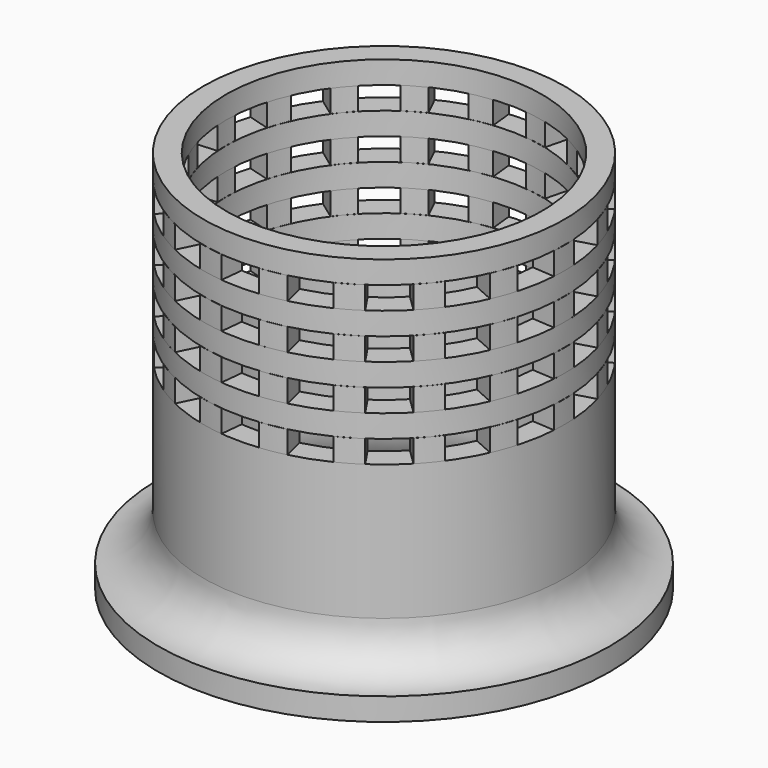
from build123d import *

# Parameters (mm, degrees)
F0_W          = 5
F0_H          = 30
F0_H_2        = 5
F2_ANGLE_BACK = 4
F2_ANGLE      = 8
F3_COUNT      = 18


# Not quite as in the source:
# - a feature names something its author has since deleted; it is built from what else it names


with BuildPart() as f1:
    # F0 (on Front) → F1 (revolve)
    with BuildSketch(Plane.XZ):
        with Locations((-37.5, 15)):
            Rectangle(F0_W, F0_H)
        with BuildLine():
            Line((-35, 0), (-40, 0))
            ThreePointArc((-40, 0), (-42.9289321881, -7.0710678119), (-50, -10))
            Line((-50, -10), (-50, -15))
            ThreePointArc((-50, -15), (-39.3933982822, -10.6066017178), (-35, 0))
        make_face()
    revolve(axis=Axis((0, 0, 67.5), (0, 0, -1)))


with BuildPart() as f1b:
    # F0 (on Front) → F1, piece 2 (revolve)
    with BuildSketch(Plane.XZ):
        with Locations((-37.5, 37.5)):
            Rectangle(F0_W, F0_H_2)
    revolve(axis=Axis((0, 0, 67.5), (0, 0, -1)))


with BuildPart() as f1c:
    # F0 (on Front) → F1, piece 3 (revolve)
    with BuildSketch(Plane.XZ):
        with Locations((-37.5, 47.5)):
            Rectangle(F0_W, F0_H_2)
    revolve(axis=Axis((0, 0, 67.5), (0, 0, -1)))


with BuildPart() as f1d:
    # F0 (on Front) → F1, piece 4 (revolve)
    with BuildSketch(Plane.XZ):
        with Locations((-37.5, 57.5)):
            Rectangle(F0_W, F0_H_2)
    revolve(axis=Axis((0, 0, 67.5), (0, 0, -1)))


with BuildPart() as f1e:
    # F0 (on Front) → F1, piece 5 (revolve)
    with BuildSketch(Plane.XZ):
        with Locations((-37.5, 67.5)):
            Rectangle(F0_W, F0_H_2)
    revolve(axis=Axis((0, 0, 67.5), (0, 0, -1)))


with BuildPart() as f2:
    # F0 (on Front) → F2 (revolve)
    with BuildSketch(Plane.XZ, mode=Mode.PRIVATE) as f2_sk:
        with Locations((-37.5, 42.5)):
            Rectangle(F0_W, F0_H_2)
    revolve(f2_sk.sketch.rotate(Axis((0, 0, 67.5), (0, 0, -1)), -F2_ANGLE_BACK), axis=Axis((0, 0, 67.5), (0, 0, -1)), revolution_arc=F2_ANGLE)


with BuildPart() as f2b:
    # F0 (on Front) → F2, piece 2 (revolve)
    with BuildSketch(Plane.XZ, mode=Mode.PRIVATE) as f2_sk:
        with Locations((-37.5, 52.5)):
            Rectangle(F0_W, F0_H_2)
    revolve(f2_sk.sketch.rotate(Axis((0, 0, 67.5), (0, 0, -1)), -F2_ANGLE_BACK), axis=Axis((0, 0, 67.5), (0, 0, -1)), revolution_arc=F2_ANGLE)


with BuildPart() as f2c:
    # F0 (on Front) → F2, piece 3 (revolve)
    with BuildSketch(Plane.XZ, mode=Mode.PRIVATE) as f2_sk:
        with Locations((-37.5, 62.5)):
            Rectangle(F0_W, F0_H_2)
    revolve(f2_sk.sketch.rotate(Axis((0, 0, 67.5), (0, 0, -1)), -F2_ANGLE_BACK), axis=Axis((0, 0, 67.5), (0, 0, -1)), revolution_arc=F2_ANGLE)


with BuildPart() as f2d:
    # F0 (on Front) → F2, piece 4 (revolve)
    with BuildSketch(Plane.XZ, mode=Mode.PRIVATE) as f2_sk:
        with Locations((-37.5, 32.5)):
            Rectangle(F0_W, F0_H_2)
    revolve(f2_sk.sketch.rotate(Axis((0, 0, 67.5), (0, 0, -1)), -F2_ANGLE_BACK), axis=Axis((0, 0, 67.5), (0, 0, -1)), revolution_arc=F2_ANGLE)


with BuildPart() as f3_1:
    # F3: instance of F2c
    add(f2c.part.rotate(Axis((0, 0, 67.5), (0, 0, -1)), 1 * 360 / F3_COUNT))


with BuildPart() as f3_2:
    # F3: instance of F2c
    add(f2c.part.rotate(Axis((0, 0, 67.5), (0, 0, -1)), 2 * 360 / F3_COUNT))


with BuildPart() as f3_3:
    # F3: instance of F2c
    add(f2c.part.rotate(Axis((0, 0, 67.5), (0, 0, -1)), 3 * 360 / F3_COUNT))


with BuildPart() as f3_4:
    # F3: instance of F2c
    add(f2c.part.rotate(Axis((0, 0, 67.5), (0, 0, -1)), 4 * 360 / F3_COUNT))


with BuildPart() as f3_5:
    # F3: instance of F2c
    add(f2c.part.rotate(Axis((0, 0, 67.5), (0, 0, -1)), 5 * 360 / F3_COUNT))


with BuildPart() as f3_6:
    # F3: instance of F2c
    add(f2c.part.rotate(Axis((0, 0, 67.5), (0, 0, -1)), 6 * 360 / F3_COUNT))


with BuildPart() as f3_7:
    # F3: instance of F2c
    add(f2c.part.rotate(Axis((0, 0, 67.5), (0, 0, -1)), 7 * 360 / F3_COUNT))


with BuildPart() as f3_8:
    # F3: instance of F2c
    add(f2c.part.rotate(Axis((0, 0, 67.5), (0, 0, -1)), 8 * 360 / F3_COUNT))


with BuildPart() as f3_9:
    # F3: instance of F2c
    add(f2c.part.rotate(Axis((0, 0, 67.5), (0, 0, -1)), 9 * 360 / F3_COUNT))


with BuildPart() as f3_10:
    # F3: instance of F2c
    add(f2c.part.rotate(Axis((0, 0, 67.5), (0, 0, -1)), 10 * 360 / F3_COUNT))


with BuildPart() as f3_11:
    # F3: instance of F2c
    add(f2c.part.rotate(Axis((0, 0, 67.5), (0, 0, -1)), 11 * 360 / F3_COUNT))


with BuildPart() as f3_12:
    # F3: instance of F2c
    add(f2c.part.rotate(Axis((0, 0, 67.5), (0, 0, -1)), 12 * 360 / F3_COUNT))


with BuildPart() as f3_13:
    # F3: instance of F2c
    add(f2c.part.rotate(Axis((0, 0, 67.5), (0, 0, -1)), 13 * 360 / F3_COUNT))


with BuildPart() as f3_14:
    # F3: instance of F2c
    add(f2c.part.rotate(Axis((0, 0, 67.5), (0, 0, -1)), 14 * 360 / F3_COUNT))


with BuildPart() as f3_15:
    # F3: instance of F2c
    add(f2c.part.rotate(Axis((0, 0, 67.5), (0, 0, -1)), 15 * 360 / F3_COUNT))


with BuildPart() as f3_16:
    # F3: instance of F2c
    add(f2c.part.rotate(Axis((0, 0, 67.5), (0, 0, -1)), 16 * 360 / F3_COUNT))


with BuildPart() as f3_17:
    # F3: instance of F2c
    add(f2c.part.rotate(Axis((0, 0, 67.5), (0, 0, -1)), 17 * 360 / F3_COUNT))


with BuildPart() as f3_18:
    # F3: instance of F2b
    add(f2b.part.rotate(Axis((0, 0, 67.5), (0, 0, -1)), 1 * 360 / F3_COUNT))


with BuildPart() as f3_19:
    # F3: instance of F2b
    add(f2b.part.rotate(Axis((0, 0, 67.5), (0, 0, -1)), 2 * 360 / F3_COUNT))


with BuildPart() as f3_20:
    # F3: instance of F2b
    add(f2b.part.rotate(Axis((0, 0, 67.5), (0, 0, -1)), 3 * 360 / F3_COUNT))


with BuildPart() as f3_21:
    # F3: instance of F2b
    add(f2b.part.rotate(Axis((0, 0, 67.5), (0, 0, -1)), 4 * 360 / F3_COUNT))


with BuildPart() as f3_22:
    # F3: instance of F2b
    add(f2b.part.rotate(Axis((0, 0, 67.5), (0, 0, -1)), 5 * 360 / F3_COUNT))


with BuildPart() as f3_23:
    # F3: instance of F2b
    add(f2b.part.rotate(Axis((0, 0, 67.5), (0, 0, -1)), 6 * 360 / F3_COUNT))


with BuildPart() as f3_24:
    # F3: instance of F2b
    add(f2b.part.rotate(Axis((0, 0, 67.5), (0, 0, -1)), 7 * 360 / F3_COUNT))


with BuildPart() as f3_25:
    # F3: instance of F2b
    add(f2b.part.rotate(Axis((0, 0, 67.5), (0, 0, -1)), 8 * 360 / F3_COUNT))


with BuildPart() as f3_26:
    # F3: instance of F2b
    add(f2b.part.rotate(Axis((0, 0, 67.5), (0, 0, -1)), 9 * 360 / F3_COUNT))


with BuildPart() as f3_27:
    # F3: instance of F2b
    add(f2b.part.rotate(Axis((0, 0, 67.5), (0, 0, -1)), 10 * 360 / F3_COUNT))


with BuildPart() as f3_28:
    # F3: instance of F2b
    add(f2b.part.rotate(Axis((0, 0, 67.5), (0, 0, -1)), 11 * 360 / F3_COUNT))


with BuildPart() as f3_29:
    # F3: instance of F2b
    add(f2b.part.rotate(Axis((0, 0, 67.5), (0, 0, -1)), 12 * 360 / F3_COUNT))


with BuildPart() as f3_30:
    # F3: instance of F2b
    add(f2b.part.rotate(Axis((0, 0, 67.5), (0, 0, -1)), 13 * 360 / F3_COUNT))


with BuildPart() as f3_31:
    # F3: instance of F2b
    add(f2b.part.rotate(Axis((0, 0, 67.5), (0, 0, -1)), 14 * 360 / F3_COUNT))


with BuildPart() as f3_32:
    # F3: instance of F2b
    add(f2b.part.rotate(Axis((0, 0, 67.5), (0, 0, -1)), 15 * 360 / F3_COUNT))


with BuildPart() as f3_33:
    # F3: instance of F2b
    add(f2b.part.rotate(Axis((0, 0, 67.5), (0, 0, -1)), 16 * 360 / F3_COUNT))


with BuildPart() as f3_34:
    # F3: instance of F2b
    add(f2b.part.rotate(Axis((0, 0, 67.5), (0, 0, -1)), 17 * 360 / F3_COUNT))


with BuildPart() as f3_35:
    # F3: instance of F2
    add(f2.part.rotate(Axis((0, 0, 67.5), (0, 0, -1)), 1 * 360 / F3_COUNT))


with BuildPart() as f3_36:
    # F3: instance of F2
    add(f2.part.rotate(Axis((0, 0, 67.5), (0, 0, -1)), 2 * 360 / F3_COUNT))


with BuildPart() as f3_37:
    # F3: instance of F2
    add(f2.part.rotate(Axis((0, 0, 67.5), (0, 0, -1)), 3 * 360 / F3_COUNT))


with BuildPart() as f3_38:
    # F3: instance of F2
    add(f2.part.rotate(Axis((0, 0, 67.5), (0, 0, -1)), 4 * 360 / F3_COUNT))


with BuildPart() as f3_39:
    # F3: instance of F2
    add(f2.part.rotate(Axis((0, 0, 67.5), (0, 0, -1)), 5 * 360 / F3_COUNT))


with BuildPart() as f3_40:
    # F3: instance of F2
    add(f2.part.rotate(Axis((0, 0, 67.5), (0, 0, -1)), 6 * 360 / F3_COUNT))


with BuildPart() as f3_41:
    # F3: instance of F2
    add(f2.part.rotate(Axis((0, 0, 67.5), (0, 0, -1)), 7 * 360 / F3_COUNT))


with BuildPart() as f3_42:
    # F3: instance of F2
    add(f2.part.rotate(Axis((0, 0, 67.5), (0, 0, -1)), 8 * 360 / F3_COUNT))


with BuildPart() as f3_43:
    # F3: instance of F2
    add(f2.part.rotate(Axis((0, 0, 67.5), (0, 0, -1)), 9 * 360 / F3_COUNT))


with BuildPart() as f3_44:
    # F3: instance of F2
    add(f2.part.rotate(Axis((0, 0, 67.5), (0, 0, -1)), 10 * 360 / F3_COUNT))


with BuildPart() as f3_45:
    # F3: instance of F2
    add(f2.part.rotate(Axis((0, 0, 67.5), (0, 0, -1)), 11 * 360 / F3_COUNT))


with BuildPart() as f3_46:
    # F3: instance of F2
    add(f2.part.rotate(Axis((0, 0, 67.5), (0, 0, -1)), 12 * 360 / F3_COUNT))


with BuildPart() as f3_47:
    # F3: instance of F2
    add(f2.part.rotate(Axis((0, 0, 67.5), (0, 0, -1)), 13 * 360 / F3_COUNT))


with BuildPart() as f3_48:
    # F3: instance of F2
    add(f2.part.rotate(Axis((0, 0, 67.5), (0, 0, -1)), 14 * 360 / F3_COUNT))


with BuildPart() as f3_49:
    # F3: instance of F2
    add(f2.part.rotate(Axis((0, 0, 67.5), (0, 0, -1)), 15 * 360 / F3_COUNT))


with BuildPart() as f3_50:
    # F3: instance of F2
    add(f2.part.rotate(Axis((0, 0, 67.5), (0, 0, -1)), 16 * 360 / F3_COUNT))


with BuildPart() as f3_51:
    # F3: instance of F2
    add(f2.part.rotate(Axis((0, 0, 67.5), (0, 0, -1)), 17 * 360 / F3_COUNT))


with BuildPart() as f3_52:
    # F3: instance of F2d
    add(f2d.part.rotate(Axis((0, 0, 67.5), (0, 0, -1)), 1 * 360 / F3_COUNT))


with BuildPart() as f3_53:
    # F3: instance of F2d
    add(f2d.part.rotate(Axis((0, 0, 67.5), (0, 0, -1)), 2 * 360 / F3_COUNT))


with BuildPart() as f3_54:
    # F3: instance of F2d
    add(f2d.part.rotate(Axis((0, 0, 67.5), (0, 0, -1)), 3 * 360 / F3_COUNT))


with BuildPart() as f3_55:
    # F3: instance of F2d
    add(f2d.part.rotate(Axis((0, 0, 67.5), (0, 0, -1)), 4 * 360 / F3_COUNT))


with BuildPart() as f3_56:
    # F3: instance of F2d
    add(f2d.part.rotate(Axis((0, 0, 67.5), (0, 0, -1)), 5 * 360 / F3_COUNT))


with BuildPart() as f3_57:
    # F3: instance of F2d
    add(f2d.part.rotate(Axis((0, 0, 67.5), (0, 0, -1)), 6 * 360 / F3_COUNT))


with BuildPart() as f3_58:
    # F3: instance of F2d
    add(f2d.part.rotate(Axis((0, 0, 67.5), (0, 0, -1)), 7 * 360 / F3_COUNT))


with BuildPart() as f3_59:
    # F3: instance of F2d
    add(f2d.part.rotate(Axis((0, 0, 67.5), (0, 0, -1)), 8 * 360 / F3_COUNT))


with BuildPart() as f3_60:
    # F3: instance of F2d
    add(f2d.part.rotate(Axis((0, 0, 67.5), (0, 0, -1)), 9 * 360 / F3_COUNT))


with BuildPart() as f3_61:
    # F3: instance of F2d
    add(f2d.part.rotate(Axis((0, 0, 67.5), (0, 0, -1)), 10 * 360 / F3_COUNT))


with BuildPart() as f3_62:
    # F3: instance of F2d
    add(f2d.part.rotate(Axis((0, 0, 67.5), (0, 0, -1)), 11 * 360 / F3_COUNT))


with BuildPart() as f3_63:
    # F3: instance of F2d
    add(f2d.part.rotate(Axis((0, 0, 67.5), (0, 0, -1)), 12 * 360 / F3_COUNT))


with BuildPart() as f3_64:
    # F3: instance of F2d
    add(f2d.part.rotate(Axis((0, 0, 67.5), (0, 0, -1)), 13 * 360 / F3_COUNT))


with BuildPart() as f3_65:
    # F3: instance of F2d
    add(f2d.part.rotate(Axis((0, 0, 67.5), (0, 0, -1)), 14 * 360 / F3_COUNT))


with BuildPart() as f3_66:
    # F3: instance of F2d
    add(f2d.part.rotate(Axis((0, 0, 67.5), (0, 0, -1)), 15 * 360 / F3_COUNT))


with BuildPart() as f3_67:
    # F3: instance of F2d
    add(f2d.part.rotate(Axis((0, 0, 67.5), (0, 0, -1)), 16 * 360 / F3_COUNT))


with BuildPart() as f3_68:
    # F3: instance of F2d
    add(f2d.part.rotate(Axis((0, 0, 67.5), (0, 0, -1)), 17 * 360 / F3_COUNT))


solid = Compound([f1.part, f1b.part, f1c.part, f1d.part, f1e.part, f2.part, f2b.part, f2c.part, f2d.part, f3_1.part, f3_2.part, f3_3.part, f3_4.part, f3_5.part, f3_6.part, f3_7.part, f3_8.part, f3_9.part, f3_10.part, f3_11.part, f3_12.part, f3_13.part, f3_14.part, f3_15.part, f3_16.part, f3_17.part, f3_18.part, f3_19.part, f3_20.part, f3_21.part, f3_22.part, f3_23.part, f3_24.part, f3_25.part, f3_26.part, f3_27.part, f3_28.part, f3_29.part, f3_30.part, f3_31.part, f3_32.part, f3_33.part, f3_34.part, f3_35.part, f3_36.part, f3_37.part, f3_38.part, f3_39.part, f3_40.part, f3_41.part, f3_42.part, f3_43.part, f3_44.part, f3_45.part, f3_46.part, f3_47.part, f3_48.part, f3_49.part, f3_50.part, f3_51.part, f3_52.part, f3_53.part, f3_54.part, f3_55.part, f3_56.part, f3_57.part, f3_58.part, f3_59.part, f3_60.part, f3_61.part, f3_62.part, f3_63.part, f3_64.part, f3_65.part, f3_66.part, f3_67.part, f3_68.part])
